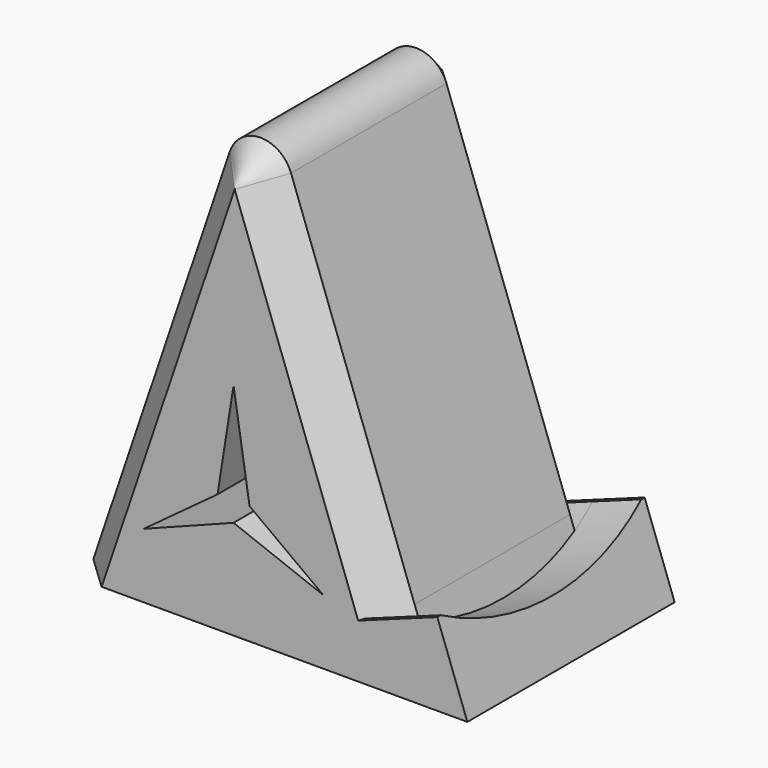
from build123d import *

# Parameters (mm, degrees)
F1_DEPTH     = 40
F4_DEPTH     = 8
F5_R         = 5
F6_T1_DEPTH  = 78.6190243925
F6_T4_ANGLE  = 141.3037112845
F6_T8_DEPTH  = 68.6190243925
F6_S9_R      = 40
F6_T10_DEPTH = 38
F6_T15_DEPTH = 55.7606094527
F6_S16_R     = 40
F6_T17_DEPTH = 31
F6_T21_DEPTH = 55.7606094527
F6_S22_R     = 40
F6_T23_DEPTH = 31
F6_T25_ANGLE = 141.3037112845
F6_T29_DEPTH = 68.6190243925
F6_S31_R     = 40
F6_T32_DEPTH = 38
F6_T36_DEPTH = 55.7606094527
F6_S37_R     = 40
F6_T38_DEPTH = 31
F6_T42_DEPTH = 55.7606094527
F6_S43_R     = 40
F6_T44_DEPTH = 31
F8_DEPTH     = 40


# Not quite as in the source:
# - a fillet or chamfer that OpenCascade refuses, or shapes differently, is made with other operations: its cross-section is extruded or revolved along the edge and cut away or added


with BuildPart() as f1:
    # F0 (on Front) → F1 (new body)
    with BuildSketch(Plane.XZ):
        Polygon((-25.644130815, 0), (0, 0), (36.0945345553, 0), (31.4589509991, 12.7361611466), (23.9414100328, 10), (0, 75.778483455), align=None)
    extrude(amount=F1_DEPTH)

    # F3 (on face) → F4 (cut, through all)
    with BuildSketch(Plane(origin=(31.8722760891, 0, 11.6005597948), x_dir=(0, 1, 0), z_dir=(0.9396926208, 0, 0.3420201433))):
        with BuildLine():
            Line((-0.635083269, 1.208481717), (-39.364916731, 1.208481717))
            ThreePointArc((-39.364916731, 1.208481717), (-20, -3.791518283), (-0.635083269, 1.208481717))
        make_face()
    extrude(amount=-F4_DEPTH, mode=Mode.SUBTRACT)

    # F5
    f5_edges = [f1.edges().sort_by_distance(p)[0] for p in [
        (0, -20, 75.778483),
    ]]
    fillet(f5_edges, radius=F5_R)

    # F6: chamfer of 5 on 2 edges, made by hand

    # F6_s2 → F6_t1 (cut)
    with BuildSketch(Plane(origin=(18.4446505209, 0, 54.5039975974), x_dir=(0, 1, 0), z_dir=(-0.3205516352, 0, -0.9472310432))):
        Polygon((-35, -24.2909167836), (-40, -19.2909167836), (-40, -24.2909167836), align=None)
        Polygon((-5, -24.2909167836), (0, -19.2909167836), (0, -24.2909167836), align=None)
    extrude(amount=F6_T1_DEPTH, mode=Mode.SUBTRACT)

    # F6_s3 → F6_t4 (revolve, cut)
    with BuildSketch(Plane(origin=(18.4446505209, 0, 54.5039975974), x_dir=(0, 1, 0), z_dir=(-0.3205516352, 0, -0.9472310432))):
        Polygon((0, -19.2909167836), (-5, -24.2909167836), (0, -24.2909167836), align=None)
    revolve(axis=Axis((0.1716952919, 0, 60.6877325166), (0, 1, 0)), revolution_arc=F6_T4_ANGLE, mode=Mode.SUBTRACT)


with BuildPart() as f6_tool6:
    # F6_s7 → F6_t8 (new body)
    with BuildSketch(Plane(origin=(3.9845118306, 0, -10.9473562821), x_dir=(0, 1, 0), z_dir=(-0.3420201433, 0, 0.9396926208))):
        Polygon((0, -20.9177677723), (-5, -25.9177677723), (0, -25.9177677723), align=None)
    extrude(amount=F6_T8_DEPTH)

    # F6_s9 → F6_t10 (intersect, symmetric)
    with BuildSketch(Plane(origin=(21.9888073264, 0, 8.0032713538), x_dir=(0, 1, 0), z_dir=(0.9396926208, 0, 0.3420201433))):
        with Locations((-20, 36.208481717)):
            Circle(F6_S9_R)
    extrude(amount=F6_T10_DEPTH, both=True, mode=Mode.INTERSECT)

    split(bisect_by=Plane(origin=(-0.4133250901, 0, 1.1356013518), x_dir=(0, 1, 0), z_dir=(0.3420201433, 0, -0.9396926208)), keep=Keep.TOP)


with BuildPart() as f1_1:
    add(f1.part)

    # F6_t5: cut F6_tool6
    add(f6_tool6.part, mode=Mode.SUBTRACT)


with BuildPart() as f6_tool13:
    # F6_s14 → F6_t15 (new body)
    with BuildSketch(Plane(origin=(-0.4133250901, 0, 1.1356013518), x_dir=(0, 1, 0), z_dir=(-0.3420201433, 0, 0.9396926208))):
        Polygon((0, -20.9177677723), (-5, -25.9177677723), (0, -25.9177677723), align=None)
    extrude(amount=F6_T15_DEPTH)

    # F6_s16 → F6_t17 (cut, symmetric)
    with BuildSketch(Plane(origin=(21.9888073264, 0, 8.0032713538), x_dir=(0, 1, 0), z_dir=(0.9396926208, 0, 0.3420201433))):
        with Locations((-20, 36.208481717)):
            Circle(F6_S16_R)
    extrude(amount=F6_T17_DEPTH, both=True, mode=Mode.SUBTRACT)


with BuildPart() as f1_2:
    add(f1_1.part)

    # F6_t12: cut F6_tool13
    add(f6_tool13.part, mode=Mode.SUBTRACT)


with BuildPart() as f6_tool19:
    # F6_s20 → F6_t21 (new body)
    with BuildSketch(Plane(origin=(-0.4133250901, 0, 1.1356013518), x_dir=(0, 1, 0), z_dir=(-0.3420201433, 0, 0.9396926208))):
        Polygon((0, -20.9177677723), (-5, -25.9177677723), (0, -25.9177677723), align=None)
    extrude(amount=F6_T21_DEPTH)

    # F6_s22 → F6_t23 (intersect, symmetric)
    with BuildSketch(Plane(origin=(21.9888073264, 0, 8.0032713538), x_dir=(0, 1, 0), z_dir=(0.9396926208, 0, 0.3420201433))):
        with Locations((-20, 36.208481717)):
            Circle(F6_S22_R)
    extrude(amount=F6_T23_DEPTH, both=True, mode=Mode.INTERSECT)


with BuildPart() as f1_3:
    add(f1_2.part)

    # F6_t18: cut F6_tool19
    add(f6_tool19.part, mode=Mode.SUBTRACT)

    # F6_s24 → F6_t25 (revolve, cut)
    with BuildSketch(Plane(origin=(18.4446505209, 0, 54.5039975974), x_dir=(0, 1, 0), z_dir=(-0.3205516352, 0, -0.9472310432))):
        Polygon((-35, -24.2909167836), (-40, -19.2909167836), (-40, -24.2909167836), align=None)
    revolve(axis=Axis((0.1716952919, -40, 60.6877325166), (0, 1, 0)), revolution_arc=F6_T25_ANGLE, mode=Mode.SUBTRACT)


with BuildPart() as f6_tool27:
    # F6_s28 → F6_t29 (new body)
    with BuildSketch(Plane(origin=(3.9845118306, 0, -10.9473562821), x_dir=(0, 1, 0), z_dir=(-0.3420201433, 0, 0.9396926208))):
        Polygon((-40, -20.9177677723), (-35, -25.9177677723), (-40, -25.9177677723), align=None)
    extrude(amount=F6_T29_DEPTH)

    split(bisect_by=Plane(origin=(-0.4133250901, 0, 1.1356013518), x_dir=(0, 1, 0), z_dir=(0.3420201433, 0, -0.9396926208)), keep=Keep.TOP)

    # F6_s31 → F6_t32 (intersect, symmetric)
    with BuildSketch(Plane(origin=(21.9888073264, 0, 8.0032713538), x_dir=(0, 1, 0), z_dir=(0.9396926208, 0, 0.3420201433))):
        with Locations((-20, 36.208481717)):
            Circle(F6_S31_R)
    extrude(amount=F6_T32_DEPTH, both=True, mode=Mode.INTERSECT)


with BuildPart() as f1_4:
    add(f1_3.part)

    # F6_t26: cut F6_tool27
    add(f6_tool27.part, mode=Mode.SUBTRACT)


with BuildPart() as f6_tool34:
    # F6_s35 → F6_t36 (new body)
    with BuildSketch(Plane(origin=(-0.4133250901, 0, 1.1356013518), x_dir=(0, 1, 0), z_dir=(-0.3420201433, 0, 0.9396926208))):
        Polygon((-40, -20.9177677723), (-35, -25.9177677723), (-40, -25.9177677723), align=None)
    extrude(amount=F6_T36_DEPTH)

    # F6_s37 → F6_t38 (cut, symmetric)
    with BuildSketch(Plane(origin=(21.9888073264, 0, 8.0032713538), x_dir=(0, 1, 0), z_dir=(0.9396926208, 0, 0.3420201433))):
        with Locations((-20, 36.208481717)):
            Circle(F6_S37_R)
    extrude(amount=F6_T38_DEPTH, both=True, mode=Mode.SUBTRACT)


with BuildPart() as f1_5:
    add(f1_4.part)

    # F6_t33: cut F6_tool34
    add(f6_tool34.part, mode=Mode.SUBTRACT)


with BuildPart() as f6_tool40:
    # F6_s41 → F6_t42 (new body)
    with BuildSketch(Plane(origin=(-0.4133250901, 0, 1.1356013518), x_dir=(0, 1, 0), z_dir=(-0.3420201433, 0, 0.9396926208))):
        Polygon((-40, -20.9177677723), (-35, -25.9177677723), (-40, -25.9177677723), align=None)
    extrude(amount=F6_T42_DEPTH)

    # F6_s43 → F6_t44 (intersect, symmetric)
    with BuildSketch(Plane(origin=(21.9888073264, 0, 8.0032713538), x_dir=(0, 1, 0), z_dir=(0.9396926208, 0, 0.3420201433))):
        with Locations((-20, 36.208481717)):
            Circle(F6_S43_R)
    extrude(amount=F6_T44_DEPTH, both=True, mode=Mode.INTERSECT)


with BuildPart() as f1_6:
    add(f1_5.part)

    # F6_t39: cut F6_tool40
    add(f6_tool40.part, mode=Mode.SUBTRACT)

    # F7 (on face) → F8 (cut, through all)
    with BuildSketch(Plane.XZ.offset(40)):
        Polygon((2.4692938483, 18.390625), (0, 34), (-2.4692938483, 18.390625), (-13.8564064606, 10), (0, 15.3219454766), (13.8564064606, 10), align=None)
    extrude(amount=-F8_DEPTH, mode=Mode.SUBTRACT)


solid = f1_6.part
